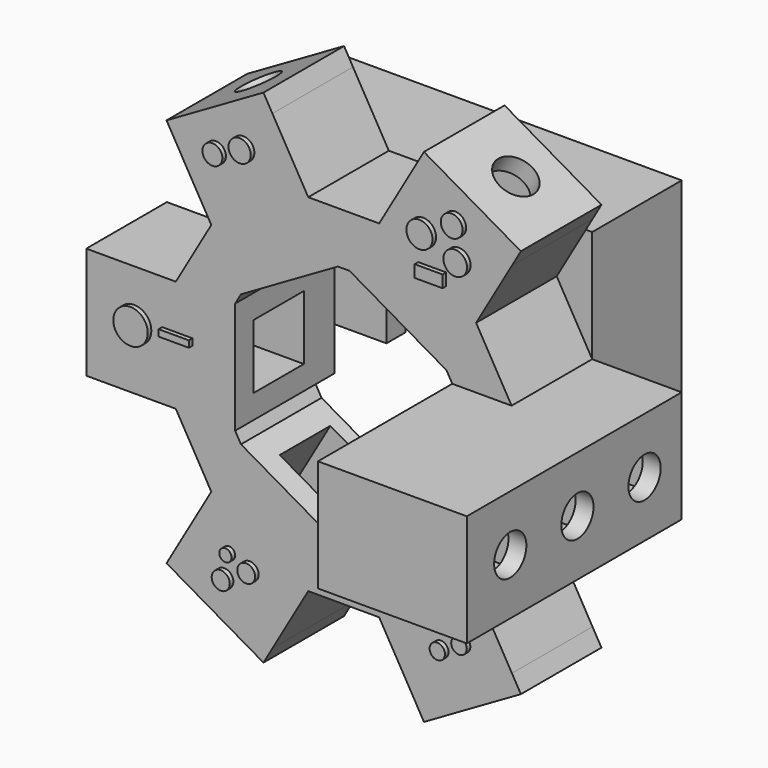
from build123d import *

# Parameters (mm, degrees)
F0_W           = 12.7
F0_H           = 3.175
F1_DEPTH       = 6.35
F2_DEPTH       = 3.683
F4_DEPTH       = 30.48
F5_W           = 7.1628
F5_H           = 7.2898
F6_DEPTH       = 38.101
F3_W           = 6.731
F3_H           = 12.7
F7_DEPTH       = 11.43
F8_W           = 3.5814
F8_H           = 3.6449
F9_DEPTH       = 12.7
F11_DEPTH      = 11.43
F12_W          = 7.2898
F12_H          = 7.1628
F13_DEPTH      = 6.731
F13_DEPTH_BACK = 31.369
F14_W          = 7.2898
F14_H          = 7.1628
F15_DEPTH      = 6.731
F15_DEPTH_BACK = 31.369
F16_W          = 7.1628
F16_H          = 7.2898
F17_DEPTH      = 8.128
F18_DEPTH      = 8.128
F19_DEPTH      = 8.128
F20_W          = 11.43
F20_H          = 12.7
F20_W_2        = 7.1628
F20_H_2        = 7.2898
F21_DEPTH      = 8.128
F22_DEPTH      = 8.128
F23_DEPTH      = 8.128
F24_W          = 12.7
F24_H          = 11.43
F24_R          = 2.286
F25_DEPTH      = 2.032
F26_W          = 12.7
F26_H          = 11.43
F26_R          = 2.286
F27_DEPTH      = 2.032
F28_W          = 11.43
F28_H          = 12.7
F28_R          = 2.286
F29_DEPTH      = 2.032
F30_W          = 12.7
F30_H          = 11.43
F30_R          = 2.286
F31_DEPTH      = 2.032
F32_W          = 12.7
F32_H          = 11.43
F32_R          = 2.286
F33_DEPTH      = 2.032
F34_W          = 30.48
F34_H          = 12.7
F34_R          = 2.286
F35_DEPTH      = 2.032
F36_R          = 1.9533985806
F36_R_2        = 1.1294229331
F36_R_3        = 1.2624825339
F36_R_4        = 1.2356748077
F36_R_5        = 1.4795101848
F36_R_6        = 1.3424473069
F36_R_7        = 0.8820699454
F36_R_8        = 0.8709860762
F36_R_9        = 1.0254141301
F36_R_10       = 0.6987220166
F36_R_11       = 1.012521994
F36_W          = 3.4493412822
F36_H          = 0.7421383634
F36_W_2        = 3.1675938517
F36_H_2        = 1.3768810313
F36_W_3        = 3.0767889693
F36_H_3        = 1.3319775462
F37_DEPTH      = 0.508


with BuildPart() as f1:
    # F0 (on Front) → F1 (new body, symmetric)
    with BuildSketch(Plane.XZ):
        with BuildLine():
            Line((0, 3.175), (0, 0))
            Line((0, 0), (13.335, 0))
            ThreePointArc((13.335, 0), (19.6211792847, -2.6038207153), (22.225, -8.89))
            Line((22.225, -8.89), (22.225, -22.225))
            Line((22.225, -22.225), (25.4, -22.225))
            Line((25.4, -22.225), (25.4, 3.175))
            Line((25.4, 3.175), (0, 3.175))
        make_face()
        with BuildLine():
            Line((13.335, 0), (0, 0))
            Line((0, 0), (0, -3.556))
            Line((0, -3.556), (11.557, -3.556))
            ThreePointArc((11.557, -3.556), (16.5859434278, -5.6390565722), (18.669, -10.668))
            Line((18.669, -10.668), (18.669, -22.225))
            Line((18.669, -22.225), (22.225, -22.225))
            Line((22.225, -22.225), (22.225, -8.89))
            ThreePointArc((22.225, -8.89), (19.6211792847, -2.6038207153), (13.335, 0))
        make_face()
        with Locations((-6.35, 1.5875)):
            Rectangle(F0_W, F0_H)
        with BuildLine():
            Line((0, -3.556), (0, 0))
            Line((0, 0), (-12.7, 0))
            Line((-12.7, 0), (-12.7, -22.225))
            Line((-12.7, -22.225), (-5.969, -22.225))
            Line((-5.969, -22.225), (-5.969, -8.636))
            ThreePointArc((-5.969, -8.636), (-4.4811024484, -5.0438975516), (-0.889, -3.556))
            Line((-0.889, -3.556), (0, -3.556))
        make_face()
    extrude(amount=F1_DEPTH, both=True)

    # F0 (on Front) → F2 (cut, symmetric)
    with BuildSketch(Plane.XZ):
        with BuildLine():
            Line((13.335, 0), (0, 0))
            Line((0, 0), (0, -3.556))
            Line((0, -3.556), (11.557, -3.556))
            ThreePointArc((11.557, -3.556), (16.5859434278, -5.6390565722), (18.669, -10.668))
            Line((18.669, -10.668), (18.669, -22.225))
            Line((18.669, -22.225), (22.225, -22.225))
            Line((22.225, -22.225), (22.225, -8.89))
            ThreePointArc((22.225, -8.89), (19.6211792847, -2.6038207153), (13.335, 0))
        make_face()
        with BuildLine():
            Line((0, -3.556), (0, 0))
            Line((0, 0), (-12.7, 0))
            Line((-12.7, 0), (-12.7, -22.225))
            Line((-12.7, -22.225), (-5.969, -22.225))
            Line((-5.969, -22.225), (-5.969, -8.636))
            ThreePointArc((-5.969, -8.636), (-4.4811024484, -5.0438975516), (-0.889, -3.556))
            Line((-0.889, -3.556), (0, -3.556))
        make_face()
    extrude(amount=F2_DEPTH, both=True, mode=Mode.SUBTRACT)

    # F3 (on face) → F4 (join)
    with BuildSketch(Plane.XZ.offset(6.35)):
        Polygon((18.669, -10.668), (18.669, -22.225), (25.4, -22.225), (25.4, -9.525), (18.669, -9.525), align=None)
    extrude(amount=F4_DEPTH)

    # F5 (on face) → F6 (cut, through all)
    with BuildSketch(Plane.YZ.offset(25.4)):
        with Locations((-11.6205, -15.875)):
            Rectangle(F5_W, F5_H)
        with Locations((-21.1455, -15.875)):
            Rectangle(F5_W, F5_H)
        with Locations((-30.6705, -15.875)):
            Rectangle(F5_W, F5_H)
    extrude(amount=-F6_DEPTH, mode=Mode.SUBTRACT)

    # F3 (on face) → F7 (join)
    with BuildSketch(Plane.XZ.offset(6.35)):
        with Locations((-9.3345, -15.875)):
            Rectangle(F3_W, F3_H)
    extrude(amount=F7_DEPTH)

    # F8 (on face) → F9 (cut)
    with BuildSketch(Plane(origin=(-12.7, 0, 0), x_dir=(0, -1, 0), z_dir=(-1, 0, 0))):
        with Locations((13.4112, -14.05255)):
            Rectangle(F8_W, F8_H)
        with Locations((9.8298, -14.05255)):
            Rectangle(F8_W, F8_H)
        Polygon((15.2019, -19.5199), (15.2019, -15.875), (11.6205, -15.875), (8.0391, -15.875), (8.0391, -19.5199), align=None)
    extrude(amount=-F9_DEPTH, mode=Mode.SUBTRACT)

    # F10 (on face) → F11 (join, through all)
    with BuildSketch(Plane.XZ.offset(6.35)):
        Polygon((-5.969, -9.525), (-5.308761314, -8.3814330508), (5.689761314, -2.0314330508), (7.010238686, -2.0314330508), (18.008761314, -8.3814330508), (18.669, -9.525), (25.4, -9.525), (21.374261314, -2.5522160579), (10.375738686, 3.7977839421), (2.324261314, 3.7977839421), (-8.674261314, -2.5522160579), (-12.7, -9.525), align=None)
        Polygon((18.008761314, -23.3685669492), (7.010238686, -29.7185669492), (5.689761314, -29.7185669492), (-5.308761314, -23.3685669492), (-5.969, -22.225), (-12.7, -22.225), (-8.674261314, -29.1977839421), (2.324261314, -35.5477839421), (10.375738686, -35.5477839421), (21.374261314, -29.1977839421), (25.4, -22.225), (18.669, -22.225), align=None)
    extrude(amount=F11_DEPTH)

    # F12 (on face) → F13 (cut, two sides)
    with BuildSketch(Plane(origin=(2.3020766425, 0, -3.9873137078), x_dir=(0.8660254038, 0, 0.5), z_dir=(0.5, 0, -0.8660254038))) as f13_sk:
        with Locations((-2.438238686, 11.6205)):
            Rectangle(F12_W, F12_H)
    extrude(amount=-F13_DEPTH, mode=Mode.SUBTRACT)
    extrude(f13_sk.sketch, amount=F13_DEPTH_BACK, mode=Mode.SUBTRACT)

    # F14 (on face) → F15 (cut, two sides)
    with BuildSketch(Plane(origin=(0.8729233575, 0, 1.5119476062), x_dir=(0.8660254038, 0, -0.5), z_dir=(-0.5, 0, -0.8660254038))) as f15_sk:
        with Locations((13.436761314, 11.6205)):
            Rectangle(F14_W, F14_H)
    extrude(amount=-F15_DEPTH, mode=Mode.SUBTRACT)
    extrude(f15_sk.sketch, amount=F15_DEPTH_BACK, mode=Mode.SUBTRACT)

    # F16 (on face) → F17 (join)
    with BuildSketch(Plane.YZ.offset(25.4)):
        Polygon((-17.78, -9.525), (-36.83, -9.525), (-36.83, -22.225), (-17.78, -22.225), (-6.35, -22.225), (-6.35, -9.525), align=None)
        with Locations((-30.6705, -15.875)):
            Rectangle(F16_W, F16_H, mode=Mode.SUBTRACT)
        with Locations((-21.1455, -15.875)):
            Rectangle(F16_W, F16_H, mode=Mode.SUBTRACT)
        with Locations((-11.6205, -15.875)):
            Rectangle(F16_W, F16_H, mode=Mode.SUBTRACT)
    extrude(amount=F17_DEPTH)

    # F18 (add): a face of the model
    f18_faces = [f1.faces().sort_by_distance(p)[0] for p in [
        (21.2262913255, -12.065, -2.4667855452),
    ]]
    extrude(f18_faces, amount=F18_DEPTH)

    # F19 (add): a face of the model
    f19_faces = [f1.faces().sort_by_distance(p)[0] for p in [
        (2.1762913255, -12.065, 3.7123534294),
    ]]
    extrude(f19_faces, amount=F19_DEPTH)

    # F20 (on face) → F21 (join)
    with BuildSketch(Plane(origin=(-12.7, 0, 0), x_dir=(0, -1, 0), z_dir=(-1, 0, 0))):
        with Locations((12.065, -15.875)):
            Rectangle(F20_W, F20_H)
        with Locations((11.6205, -15.875)):
            Rectangle(F20_W_2, F20_H_2, mode=Mode.SUBTRACT)
    extrude(amount=F21_DEPTH)

    # F22 (add): a face of the model
    f22_faces = [f1.faces().sort_by_distance(p)[0] for p in [
        (-8.5262913255, -12.065, -29.2832144548),
    ]]
    extrude(f22_faces, amount=F22_DEPTH)

    # F23 (add): a face of the model
    f23_faces = [f1.faces().sort_by_distance(p)[0] for p in [
        (10.5237086745, -12.065, -35.4623534294),
    ]]
    extrude(f23_faces, amount=F23_DEPTH)

    # F24 (on face) → F25 (join)
    with BuildSketch(Plane(origin=(8.3024233575, 0, 14.3802190811), x_dir=(0.8660254038, 0, -0.5), z_dir=(0.5, 0, 0.8660254038))):
        with Locations((13.436761314, -12.065)):
            Rectangle(F24_W, F24_H)
        with Locations((13.436761314, -11.6205)):
            Circle(F24_R, mode=Mode.SUBTRACT)
    extrude(amount=F25_DEPTH)

    # F26 (on face) → F27 (join)
    with BuildSketch(Plane(origin=(-5.1274233575, 0, 8.880957767), x_dir=(0.8660254038, 0, 0.5), z_dir=(-0.5, 0, 0.8660254038))):
        with Locations((-2.438238686, -12.065)):
            Rectangle(F26_W, F26_H)
        with Locations((-2.4382386859, -11.6205)):
            Circle(F26_R, mode=Mode.SUBTRACT)
    extrude(amount=F27_DEPTH)

    # F28 (on face) → F29 (join)
    with BuildSketch(Plane(origin=(-20.828, 0, 0), x_dir=(0, -1, 0), z_dir=(-1, 0, 0))):
        with Locations((12.065, -15.875)):
            Rectangle(F28_W, F28_H)
        with Locations((11.6205, -15.875)):
            Circle(F28_R, mode=Mode.SUBTRACT)
    extrude(amount=F29_DEPTH)

    # F30 (on face) → F31 (join)
    with BuildSketch(Plane(origin=(-18.8755766425, 0, -32.693457767), x_dir=(0.8660254038, 0, -0.5), z_dir=(-0.5, 0, -0.8660254038))):
        with Locations((13.436761314, 12.065)):
            Rectangle(F30_W, F30_H)
        with Locations((13.436761314, 11.6205)):
            Circle(F30_R, mode=Mode.SUBTRACT)
    extrude(amount=F31_DEPTH)

    # F32 (on face) → F33 (join)
    with BuildSketch(Plane(origin=(22.0505766425, 0, -38.1927190811), x_dir=(0.8660254038, 0, 0.5), z_dir=(0.5, 0, -0.8660254038))):
        with Locations((-2.438238686, 12.065)):
            Rectangle(F32_W, F32_H)
        with Locations((-2.4382386859, 11.6205)):
            Circle(F32_R, mode=Mode.SUBTRACT)
    extrude(amount=F33_DEPTH)

    # F34 (on face) → F35 (join)
    with BuildSketch(Plane.YZ.offset(33.528)):
        with Locations((-21.59, -15.875)):
            Rectangle(F34_W, F34_H)
        with Locations((-30.6705, -15.875)):
            Circle(F34_R, mode=Mode.SUBTRACT)
        with Locations((-21.1455, -15.875)):
            Circle(F34_R, mode=Mode.SUBTRACT)
        with Locations((-11.6205, -15.875)):
            Circle(F34_R, mode=Mode.SUBTRACT)
    extrude(amount=F35_DEPTH)

    # F36 (on face) → F37 (join)
    with BuildSketch(Plane.XZ.offset(17.78)):
        with Locations((-17.4339655787, -15.3335016221)):
            Circle(F36_R)
        with Locations((-8.1460978836, 4.867112264)):
            Circle(F36_R_2)
        with Locations((-5.0520505756, 6.2466020445)):
            Circle(F36_R_3)
        with Locations((19.006319344, 6.5597151406)):
            Circle(F36_R_4)
        with Locations((15.3510505334, 4.5153293759)):
            Circle(F36_R_5)
        with Locations((19.4071084261, 2.9789232649)):
            Circle(F36_R_6)
        with Locations((19.83676292, -35.1207405329)):
            Circle(F36_R_7)
        with Locations((17.3755344003, -36.4661067724)):
            Circle(F36_R_8)
        with Locations((-7.1977977641, -37.3765304685)):
            Circle(F36_R_9)
        with Locations((-6.6677220166, -34.6863158047)):
            Circle(F36_R_10)
        with Locations((-4.3116188608, -35.7335619628)):
            Circle(F36_R_11)
        with Locations((-12.5252148136, -14.9380327202)):
            Rectangle(F36_W, F36_H)
        with Locations((16.394414939, 0.6884405157)):
            Rectangle(F36_W_2, F36_H_2)
        with Locations((17.0683967881, -32.4682071805)):
            Rectangle(F36_W_3, F36_H_3)
    extrude(amount=F37_DEPTH)


solid = f1.part
